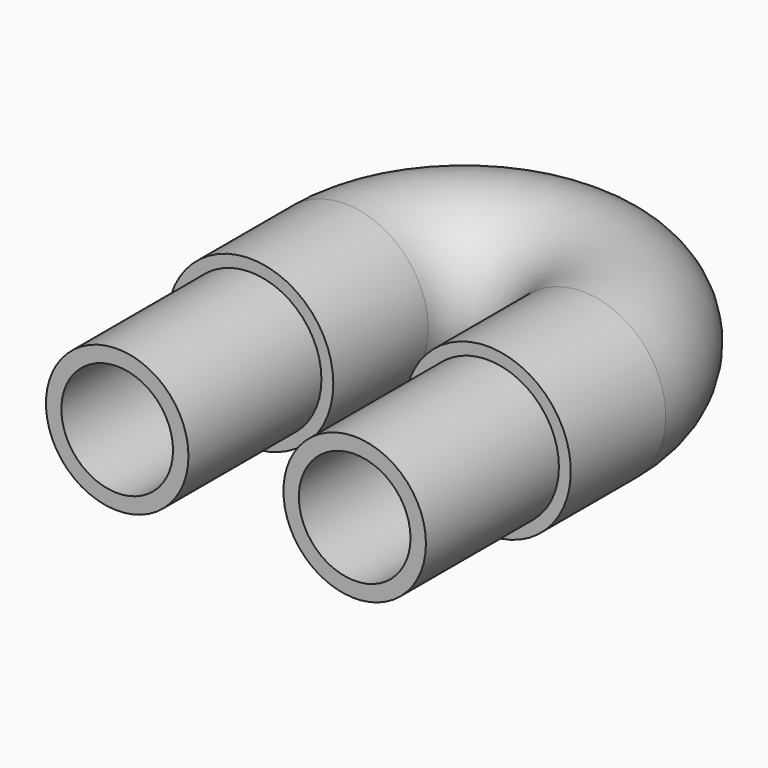
from build123d import *
from build123d import SkipClean  # not in build123d's __all__

# Parameters (mm, degrees)
F0_R     = 8.89
F0_R_2   = 5.969
F3_R     = 7.62
F3_R_2   = 5.969
F4_R     = 7.62
F4_R_2   = 5.969
F5_DEPTH = 17.78


with BuildPart() as f2:
    # F2: sweep along a path in F1
    with BuildLine(Plane.XY) as f2_path:
        Line((0, 0), (0, 12.7))
        ThreePointArc((0, 12.7), (12.7, 25.4), (25.4, 12.7))
        Line((25.4, 12.7), (25.4, 0))
    # F0 (on Front) → F2 (sweep)
    with BuildSketch(Plane.XZ):
        Circle(F0_R)
        Circle(F0_R_2, mode=Mode.SUBTRACT)
    sweep(path=f2_path.line)

    # F3 (on face) + F4 (on face) → F5 (join)
    with BuildSketch(Plane.XZ):
        Circle(F3_R)
        Circle(F3_R_2, mode=Mode.SUBTRACT)
    with BuildSketch(Plane.XZ):
        with Locations((25.4, 0)):
            Circle(F4_R)
        with Locations((25.4, 0)):
            Circle(F4_R_2, mode=Mode.SUBTRACT)
    with SkipClean():  # cleaning this boolean's faces spoils the solid; the shape is the same uncleaned
        extrude(amount=F5_DEPTH)


solid = f2.part
